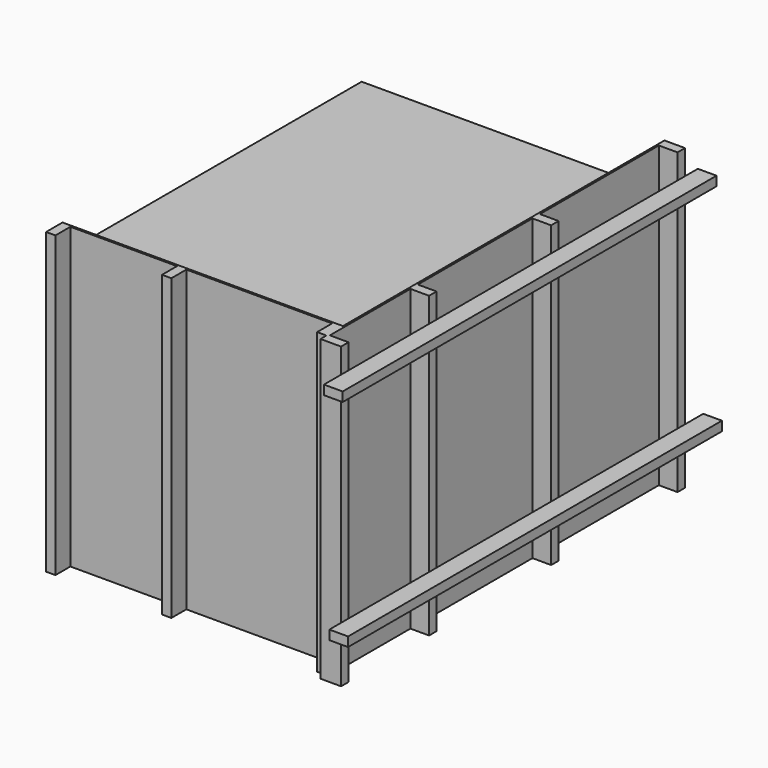
from build123d import *

# Parameters (mm, degrees)
F0_W      = 1500
F0_H      = 2000
F1_DEPTH  = 1300
F2_W      = 2300
F2_H      = 1600
F2_W_2    = 2000
F2_H_2    = 1300
F3_DEPTH  = 10
F4_W      = 50
F4_H      = 1600
F5_DEPTH  = 100
F6_W      = 114.3861696124
F6_H      = 50
F6_W_2    = 50
F6_W_3    = 2335.6138303876
F6_W_4    = 2371.7742994428
F6_W_5    = 78.2257005572
F7_DEPTH  = 100
F8_W      = 1500
F8_H      = 150
F8_H_2    = 1300
F9_DEPTH  = 10
F10_W     = 50
F10_H     = 1600
F11_DEPTH = 100


with BuildPart() as f1:
    # F0 (on Top) → F1 (new body)
    with BuildSketch(Plane.XY):
        with Locations((-698.2090473175, 942.9008886218)):
            Rectangle(F0_W, F0_H)
    extrude(amount=F1_DEPTH)

    # F2 (on face) → F3 (join)
    with BuildSketch(Plane.YZ.offset(51.7909526825)):
        with Locations((942.9008886218, 650)):
            Rectangle(F2_W, F2_H)
        with Locations((942.9008886218, 650)):
            Rectangle(F2_W_2, F2_H_2, mode=Mode.SUBTRACT)
        with Locations((942.9008886218, 650)):
            Rectangle(F2_W_2, F2_H_2)
    extrude(amount=F3_DEPTH)

    # F4 (on face) → F5 (join)
    with BuildSketch(Plane.YZ.offset(61.7909526825)):
        with Locations((-182.0991113782, 650)):
            Rectangle(F4_W, F4_H)
        with Locations((406.4638853073, 650)):
            Rectangle(F4_W, F4_H)
        with Locations((1222.7266073227, 650)):
            Rectangle(F4_W, F4_H)
        with Locations((2067.9008886218, 650)):
            Rectangle(F4_W, F4_H)
    extrude(amount=F5_DEPTH)

    # F6 (on face) → F7 (join)
    with BuildSketch(Plane.YZ.offset(161.7909526825)):
        with Locations((-264.2921961844, 1292.5743103027)):
            Rectangle(F6_W, F6_H)
        with Locations((-182.0991113782, 1292.5743103027)):
            Rectangle(F6_W_2, F6_H)
        with Locations((1010.7078038156, 1292.5743103027)):
            Rectangle(F6_W_3, F6_H)
        with Locations((1028.7880383432, 124.1379097104)):
            Rectangle(F6_W_4, F6_H)
        with Locations((-182.0991113782, 124.1379097104)):
            Rectangle(F6_W_2, F6_H)
        with Locations((-246.2119616568, 124.1379097104)):
            Rectangle(F6_W_5, F6_H)
    extrude(amount=F7_DEPTH)

    # F8 (on face) → F9 (join)
    with BuildSketch(Plane.XZ.offset(57.0991113782)):
        with Locations((-698.2090473175, 1375)):
            Rectangle(F8_W, F8_H)
        with Locations((-698.2090473175, 650)):
            Rectangle(F8_W, F8_H_2)
        with Locations((-698.2090473175, -75)):
            Rectangle(F8_W, F8_H)
    extrude(amount=F9_DEPTH)

    # F10 (on face) → F11 (join)
    with BuildSketch(Plane.XZ.offset(67.0991113782)):
        with Locations((26.7909526825, 650)):
            Rectangle(F10_W, F10_H)
        with Locations((-802.9731273651, 650)):
            Rectangle(F10_W, F10_H)
        with Locations((-1423.2090473175, 650)):
            Rectangle(F10_W, F10_H)
    extrude(amount=F11_DEPTH)


solid = f1.part
